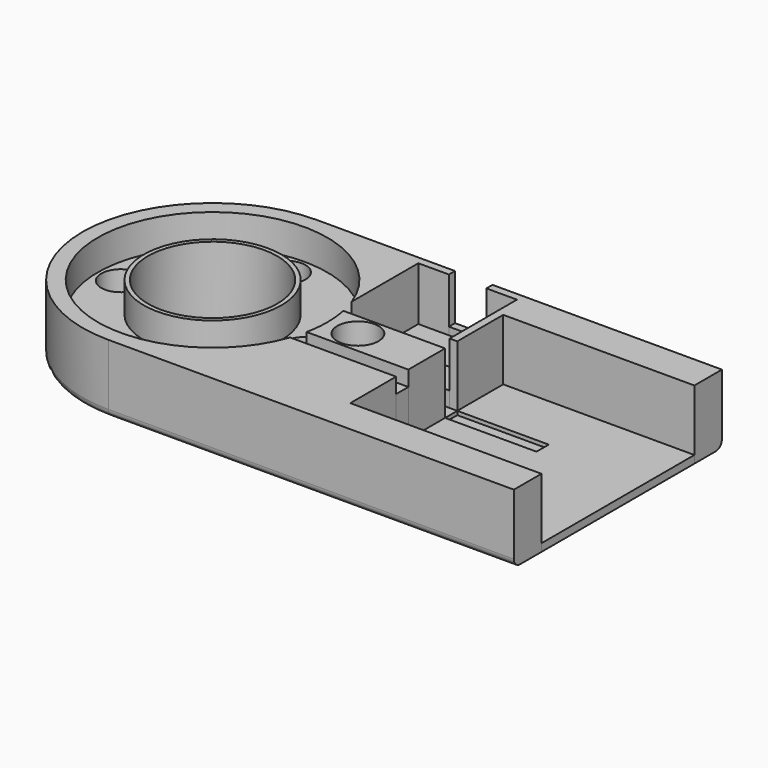
from build123d import *

# Parameters (mm, degrees)
F1_DEPTH = 9
F0_R     = 2.7
F0_R_2   = 9
F0_R_3   = 8.45
F2_DEPTH = 1
F3_DEPTH = 2
F0_W     = 11.9553784338
F0_H     = 2
F4_DEPTH = 0.5
F5_DEPTH = 7
F0_R_4   = 2.55
F6_DEPTH = 5
F7_DEPTH = 3
F0_W_2   = 4.9
F0_H_2   = 1
F9_R     = 0.99999
F9_2_R   = 0.99999
F9_3_R   = 0.99999


# Not quite as in the source:
# - a fillet or chamfer that OpenCascade refuses, or shapes differently, is made with other operations: its cross-section is extruded or revolved along the edge and cut away or added
# - a fillet or chamfer is up to 0.001 mm smaller than in the source, because OpenCascade refuses the exact size


with BuildPart() as f1:
    # F0 (on Top) → F1 (new body)
    with BuildSketch(Plane.XY):
        with BuildLine():
            Line((10.1853074353, 17), (-7.9146925647, 17))
            ThreePointArc((-7.9146925647, 17), (-24.9146925647, 0), (-7.9146925647, -17))
            Line((-7.9146925647, -17), (45.0853074353, -17))
            Line((45.0853074353, -17), (45.0853074353, -12.5))
            Line((45.0853074353, -12.5), (20.0853074353, -12.5))
            Line((20.0853074353, -12.5), (20.0853074353, -5))
            Line((20.0853074353, -5), (6.227443059, -5))
            ThreePointArc((6.227443059, -5), (-22.9145624885, -0.0624681581), (6.1853074353, 5.1176166328))
            Line((6.1853074353, 5.1176166328), (6.1853074353, 6))
            Line((6.1853074353, 6), (6.1853074353, 9.1))
            Line((6.1853074353, 9.1), (6.1853074353, 16))
            Line((6.1853074353, 16), (10.1853074353, 16))
            Line((10.1853074353, 16), (10.1853074353, 17))
        make_face()
    extrude(amount=F1_DEPTH)

    # F9 (radius 1 in the source; OpenCascade refuses exactly that, so slightly less here)
    f9_edges = [f1.edges().sort_by_distance(p)[0] for p in [
        (1.135307, 17, 0),
        (-24.914693, 0, 0),
        (18.585307, -17, 0),
    ]]
    fillet(f9_edges, radius=F9_R)


with BuildPart() as f1b:
    # F0 (on Top) → F1, piece 2 (new body)
    with BuildSketch(Plane.XY):
        Polygon((45.0853074353, 17), (15.0853074353, 17), (15.0853074353, 16), (19.0853074353, 16), (19.0853074353, 9.1), (19.0853074353, 6), (19.0853074353, 5), (20.0853074353, 5), (20.0853074353, 12.5), (45.0853074353, 12.5), align=None)
    extrude(amount=F1_DEPTH)

    # F9#2 (radius 1 in the source; OpenCascade refuses exactly that, so slightly less here)
    f9_2_edges = [f1b.edges().sort_by_distance(p)[0] for p in [
        (30.085307, 17, 0),
    ]]
    fillet(f9_2_edges, radius=F9_2_R)


with BuildPart() as f1c:
    # F0 (on Top) → F1, piece 3 (new body)
    with BuildSketch(Plane.XY):
        with BuildLine():
            Line((6.782245892, -3), (20.0853074353, -3))
            Line((20.0853074353, -3), (20.0853074353, 3))
            Line((20.0853074353, 3), (6.782245892, 3))
            ThreePointArc((6.782245892, 3), (7.0093497304, 1.5076344301), (7.0853074353, 0))
            ThreePointArc((7.0853074353, 0), (7.0093497304, -1.5076344301), (6.782245892, -3))
        make_face()
        with Locations((11.0853074353, 0)):
            Circle(F0_R, mode=Mode.SUBTRACT)
    extrude(amount=F1_DEPTH)


with BuildPart() as f1d:
    # F0 (on Top) → F1, piece 4 (new body)
    with BuildSketch(Plane.XY):
        with Locations((-7.9146925647, 0)):
            Circle(F0_R_2)
        with Locations((-7.9146925647, 0)):
            Circle(F0_R_3, mode=Mode.SUBTRACT)
    extrude(amount=F1_DEPTH)


with BuildPart() as f2:
    # F0 (on Top) → F2 (new body)
    with BuildSketch(Plane.XY):
        Polygon((20.0853074353, -12.5), (45.0853074353, -12.5), (45.0853074353, 12.5), (20.0853074353, 12.5), (20.0853074353, 5), (32.0406858691, 5), (32.0406858691, 3), (20.0853074353, 3), (20.0853074353, -3), (20.0853074353, -5), align=None)
    extrude(amount=F2_DEPTH)

    # F0 (on Top) → F4 (join)
    with BuildSketch(Plane.XY):
        with Locations((26.0629966522, 4)):
            Rectangle(F0_W, F0_H)
    extrude(amount=F4_DEPTH)


with BuildPart() as f2b:
    # F0 (on Top) → F2, piece 2 (new body)
    with BuildSketch(Plane.XY):
        with BuildLine():
            Line((20.0853074353, 3), (20.0853074353, 5))
            Line((20.0853074353, 5), (19.0853074353, 5))
            Line((19.0853074353, 5), (6.227443059, 5))
            ThreePointArc((6.227443059, 5), (6.5394780602, 4.0096074055), (6.782245892, 3))
            Line((6.782245892, 3), (20.0853074353, 3))
        make_face()
    extrude(amount=F2_DEPTH)


with BuildPart() as f3:
    # F0 (on Top) → F3 (new body)
    with BuildSketch(Plane.XY):
        Polygon((15.0853074353, 16), (10.1853074353, 16), (6.1853074353, 16), (6.1853074353, 9.1), (19.0853074353, 9.1), (19.0853074353, 16), align=None)
    extrude(amount=F3_DEPTH)


with BuildPart() as f4:
    # F0 (on Top) → F4, piece 2 (new body)
    with BuildSketch(Plane.XY):
        with Locations((11.0853074353, 0)):
            Circle(F0_R)
    extrude(amount=F4_DEPTH)


with BuildPart() as f5:
    # F0 (on Top) → F5 (new body)
    with BuildSketch(Plane.XY):
        with BuildLine():
            Line((6.227443059, -5), (20.0853074353, -5))
            Line((20.0853074353, -5), (20.0853074353, -3))
            Line((20.0853074353, -3), (6.782245892, -3))
            ThreePointArc((6.782245892, -3), (6.5394780602, -4.0096074055), (6.227443059, -5))
        make_face()
    extrude(amount=F5_DEPTH)


with BuildPart() as f6:
    # F0 (on Top) → F6 (new body)
    with BuildSketch(Plane.XY):
        with BuildLine():
            ThreePointArc((6.227443059, 5), (6.2064977026, 5.0588521855), (6.1853074353, 5.1176166328))
            ThreePointArc((6.1853074353, 5.1176166328), (-22.9145624885, -0.0624681581), (6.227443059, -5))
            ThreePointArc((6.227443059, -5), (6.5394780602, -4.0096074055), (6.782245892, -3))
            ThreePointArc((6.782245892, -3), (7.0093497304, -1.5076344301), (7.0853074353, 0))
            ThreePointArc((7.0853074353, 0), (7.0093497304, 1.5076344301), (6.782245892, 3))
            ThreePointArc((6.782245892, 3), (6.5394780602, 4.0096074055), (6.227443059, 5))
        make_face()
        with Locations((-7.9146925647, -12)):
            Circle(F0_R_4, mode=Mode.SUBTRACT)
        with Locations((-19.9146925647, 0)):
            Circle(F0_R_4, mode=Mode.SUBTRACT)
        with Locations((-7.9146925647, 0)):
            Circle(F0_R_2, mode=Mode.SUBTRACT)
        with Locations((4.0853074353, 0)):
            Circle(F0_R_4, mode=Mode.SUBTRACT)
        with Locations((-7.9146925647, 12)):
            Circle(F0_R_4, mode=Mode.SUBTRACT)
    extrude(amount=F6_DEPTH)

    # F8: fillet of radius 0.5 on 4 edges, made by hand

    # F8_s1 → F8_t2 (revolve, cut)
    with BuildSketch(Plane.XZ):
        with BuildLine():
            ThreePointArc((-17.3646925647, 0.5), (-17.2182459553, 0.1464466094), (-16.8646925647, 0))
            Line((-16.8646925647, 0), (-17.3646925647, 0))
            Line((-17.3646925647, 0), (-17.3646925647, 0.5))
        make_face()
    revolve(axis=Axis((-19.9146925647, 0, 0), (0, 0, 1)), mode=Mode.SUBTRACT)

    # F8_s3 → F8_t4 (revolve, cut)
    with BuildSketch(Plane.XZ.offset(12)):
        with BuildLine():
            ThreePointArc((-5.3646925647, 0.5), (-5.2182459553, 0.1464466094), (-4.8646925647, 0))
            Line((-4.8646925647, 0), (-5.3646925647, 0))
            Line((-5.3646925647, 0), (-5.3646925647, 0.5))
        make_face()
    revolve(axis=Axis((-7.9146925647, -12, 0), (0, 0, 1)), mode=Mode.SUBTRACT)

    # F8_s5 → F8_t6 (revolve, cut)
    with BuildSketch(Plane.XZ):
        with BuildLine():
            ThreePointArc((6.6353074353, 0.5), (6.7817540447, 0.1464466094), (7.1353074353, 0))
            Line((7.1353074353, 0), (6.6353074353, 0))
            Line((6.6353074353, 0), (6.6353074353, 0.5))
        make_face()
    revolve(axis=Axis((4.0853074353, 0, 0), (0, 0, 1)), mode=Mode.SUBTRACT)

    # F8_s7 → F8_t8 (revolve, cut)
    with BuildSketch(Plane.XZ.offset(-12)):
        with BuildLine():
            ThreePointArc((-5.3646925647, 0.5), (-5.2182459553, 0.1464466094), (-4.8646925647, 0))
            Line((-4.8646925647, 0), (-5.3646925647, 0))
            Line((-5.3646925647, 0), (-5.3646925647, 0.5))
        make_face()
    revolve(axis=Axis((-7.9146925647, 12, 0), (0, 0, 1)), mode=Mode.SUBTRACT)


with BuildPart() as f7:
    # F0 (on Top) → F7 (new body)
    with BuildSketch(Plane.XY):
        with BuildLine():
            Line((19.0853074353, 9.1), (6.1853074353, 9.1))
            Line((6.1853074353, 9.1), (6.1853074353, 6))
            Line((6.1853074353, 6), (6.1853074353, 5.1176166328))
            ThreePointArc((6.1853074353, 5.1176166328), (6.2064977026, 5.0588521855), (6.227443059, 5))
            Line((6.227443059, 5), (19.0853074353, 5))
            Line((19.0853074353, 5), (19.0853074353, 6))
            Line((19.0853074353, 6), (19.0853074353, 9.1))
        make_face()
    extrude(amount=F7_DEPTH)


with BuildPart() as f7b:
    # F0 (on Top) → F7, piece 2 (new body)
    with BuildSketch(Plane.XY):
        with Locations((12.6353074353, 16.5)):
            Rectangle(F0_W_2, F0_H_2)
    extrude(amount=F7_DEPTH)

    # F9#3 (radius 1 in the source; OpenCascade refuses exactly that, so slightly less here)
    f9_3_edges = [f7b.edges().sort_by_distance(p)[0] for p in [
        (12.635307, 17, 0),
    ]]
    fillet(f9_3_edges, radius=F9_3_R)


solid = Compound([f1.part, f1b.part, f1c.part, f1d.part, f2.part, f2b.part, f3.part, f4.part, f5.part, f6.part, f7.part, f7b.part])
